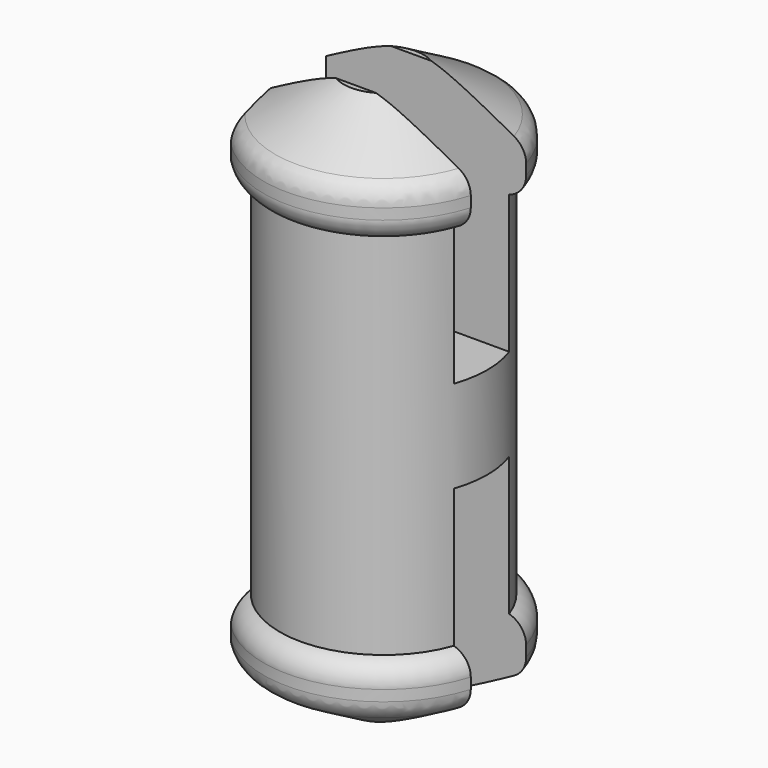
from build123d import *

# Parameters (mm, degrees)
F0_R         = 2.6
F1_DEPTH     = 2
F2_R         = 2.25
F3_DEPTH     = 8
F4_R         = 2.6
F5_DEPTH     = 2
F8_DEPTH     = 5
F10_DEPTH    = 5
F11_C1_SIZE2 = 1
F11_C1_SIZE  = 1.7320508076
F11_C2_SIZE2 = 1
F11_C2_SIZE  = 1.7320508076
F12_C1_SIZE2 = 1
F12_C1_SIZE  = 1.7320508076
F12_C2_SIZE2 = 1
F12_C2_SIZE  = 1.7320508076
F13_R        = 0.5
F15_DEPTH    = 25


# Not quite as in the source:
# - a fillet or chamfer that OpenCascade refuses, or shapes differently, is made with other operations: its cross-section is extruded or revolved along the edge and cut away or added


with BuildPart() as f1:
    # F0 (on Top) → F1 (new body)
    with BuildSketch(Plane.XY):
        Circle(F0_R)
    extrude(amount=F1_DEPTH)

    # F2 (on face) → F3 (join)
    with BuildSketch(Plane.XY.offset(2)):
        Circle(F2_R)
    extrude(amount=F3_DEPTH)

    # F4 (on face) → F5 (join)
    with BuildSketch(Plane.XY.offset(10)):
        Circle(F4_R)
    extrude(amount=F5_DEPTH)

    # F6: fillet of radius 0.5 on 2 edges, made by hand

    # F6_s1 → F6_t2 (revolve, cut)
    with BuildSketch(Plane.XZ):
        with BuildLine():
            ThreePointArc((2.25, 2), (2.5031128874, 1.8188343884), (2.6, 1.5230303993))
            Line((2.6, 1.5230303993), (2.6, 2))
            Line((2.6, 2), (2.25, 2))
        make_face()
    revolve(axis=Axis((0, 0, 2), (0, 0, 1)), mode=Mode.SUBTRACT)

    # F6_s3 → F6_t4 (revolve, cut)
    with BuildSketch(Plane.XZ):
        with BuildLine():
            ThreePointArc((2.6, 10.4769696007), (2.5031128874, 10.1811656116), (2.25, 10))
            Line((2.25, 10), (2.6, 10))
            Line((2.6, 10), (2.6, 10.4769696007))
        make_face()
    revolve(axis=Axis((0, 0, 10), (0, 0, 1)), mode=Mode.SUBTRACT)

    # F7 (on face) → F8 (cut)
    with BuildSketch(Plane(origin=(0, 0, 0), x_dir=(1, 0, 0), z_dir=(0, 0, -1))):
        with BuildLine():
            ThreePointArc((-2.4894778569, 0.75), (-2.6, 0), (-2.4894778569, -0.75))
            Line((-2.4894778569, -0.75), (2.4894778569, -0.75))
            ThreePointArc((2.4894778569, -0.75), (2.6, 0), (2.4894778569, 0.75))
            Line((2.4894778569, 0.75), (-2.4894778569, 0.75))
        make_face()
    extrude(amount=-F8_DEPTH, mode=Mode.SUBTRACT)

    # F9 (on face) → F10 (cut)
    with BuildSketch(Plane.XY.offset(12)):
        with BuildLine():
            ThreePointArc((-2.4894778569, 0.75), (-2.6, 0), (-2.4894778569, -0.75))
            Line((-2.4894778569, -0.75), (2.4894778569, -0.75))
            ThreePointArc((2.4894778569, -0.75), (2.6, 0), (2.4894778569, 0.75))
            Line((2.4894778569, 0.75), (-2.4894778569, 0.75))
        make_face()
    extrude(amount=-F10_DEPTH, mode=Mode.SUBTRACT)

    # F11: chamfer of 1 x 1.7320508076 on 2 edges, made by hand

    # F11_c1
    f11_c1_edges = [f1.edges().sort_by_distance(p)[0] for p in [
        (0, 2.6, 0),
    ]]
    f11_c1_side = f1.faces().sort_by_distance((0, 2.58, 0))[0]
    chamfer(f11_c1_edges, length=F11_C1_SIZE, length2=F11_C1_SIZE2, reference=f11_c1_side)

    # F11_c2
    f11_c2_edges = [f1.edges().sort_by_distance(p)[0] for p in [
        (0, -2.6, 0),
    ]]
    f11_c2_side = f1.faces().sort_by_distance((0, -2.58, 0))[0]
    chamfer(f11_c2_edges, length=F11_C2_SIZE, length2=F11_C2_SIZE2, reference=f11_c2_side)

    # F12: chamfer of 1 x 1.7320508076 on 2 edges, made by hand

    # F12_c1
    f12_c1_edges = [f1.edges().sort_by_distance(p)[0] for p in [
        (0, -2.6, 12),
    ]]
    f12_c1_side = f1.faces().sort_by_distance((0, -2.58, 12))[0]
    chamfer(f12_c1_edges, length=F12_C1_SIZE, length2=F12_C1_SIZE2, reference=f12_c1_side)

    # F12_c2
    f12_c2_edges = [f1.edges().sort_by_distance(p)[0] for p in [
        (0, 2.6, 12),
    ]]
    f12_c2_side = f1.faces().sort_by_distance((0, 2.58, 12))[0]
    chamfer(f12_c2_edges, length=F12_C2_SIZE, length2=F12_C2_SIZE2, reference=f12_c2_side)

    # F13
    f13_edges = [f1.edges().sort_by_distance(p)[0] for p in [
        (0, -2.6, 11),
        (0, 2.6, 11),
        (0, -2.6, 1),
        (0, 2.6, 1),
    ]]
    fillet(f13_edges, radius=F13_R)

    # F14 (on face) → F15 (cut)
    with BuildSketch(Plane.XY.offset(12)):
        with BuildLine():
            Line((-1.85, -1.8268825906), (-1.85, 1.8268825906))
            ThreePointArc((-1.85, 1.8268825906), (-2.6, 0), (-1.85, -1.8268825906))
        make_face()
    extrude(amount=-F15_DEPTH, mode=Mode.SUBTRACT)


solid = f1.part
